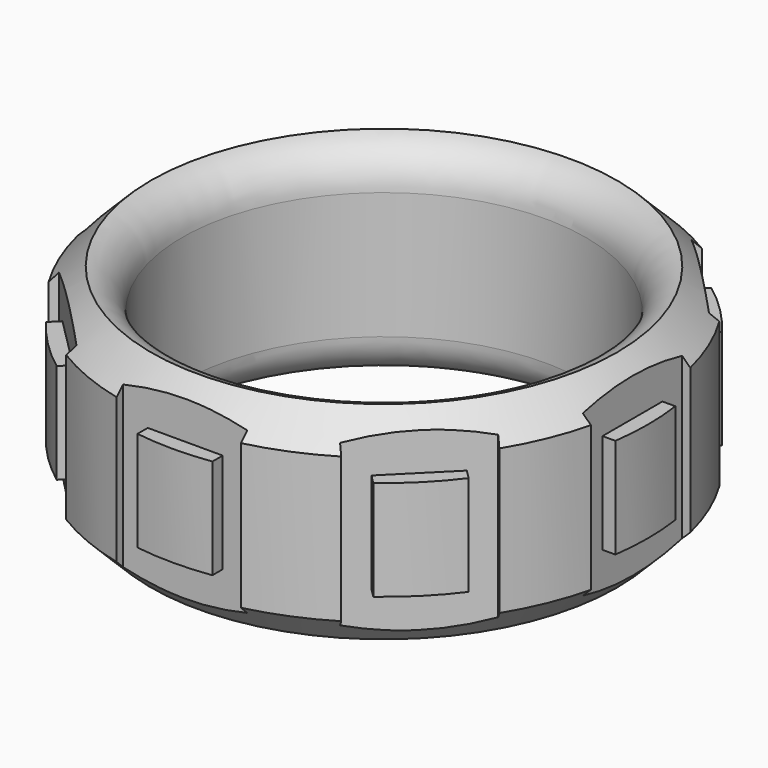
from build123d import *

# Parameters (mm, degrees)
F0_R            = 12.75
F0_R_2          = 9.75
F1_DEPTH        = 10
F2_SIZE         = 1.5
F4_W            = 6
F4_H            = 10
F4_W_2          = 3.618944902
F4_H_2          = 4.83566802
F5_DEPTH        = 2
F5_COPIES_COUNT = 8


# Not quite as in the source:
# - a fillet or chamfer that OpenCascade refuses, or shapes differently, is made with other operations: its cross-section is extruded or revolved along the edge and cut away or added
# - a pattern or mirror of a feature is missing from the dataset's text; its kind, count and spacing are read off the source's solid


with BuildPart() as f1:
    # F0 (on Top) → F1 (new body)
    with BuildSketch(Plane.XY):
        Circle(F0_R)
        Circle(F0_R_2, mode=Mode.SUBTRACT)
    extrude(amount=F1_DEPTH)

    # F2
    f2_edges = [f1.edges().sort_by_distance(p)[0] for p in [
        (-12.75, 0, 10),
        (-12.75, 0, 0),
    ]]
    chamfer(f2_edges, length=F2_SIZE)

    # F4 (on offset) → F5 (cut)
    with BuildSketch(Plane.YZ.offset(14)):
        with Locations((0, 5.0058439374)):
            Rectangle(F4_W, F4_H)
        with Locations((0, 5.0058439374)):
            Rectangle(F4_W_2, F4_H_2, mode=Mode.SUBTRACT)
    f5 = extrude(amount=-F5_DEPTH, mode=Mode.SUBTRACT)

    # F5_copies: F5 ×8 about axis
    f5_copies_axis = Axis((0, 0, 0), (0, 0, 1))
    for i in range(1, F5_COPIES_COUNT):
        add(f5.rotate(f5_copies_axis, i * 360 / F5_COPIES_COUNT), mode=Mode.SUBTRACT)

    # F6: fillet of radius 2 on 2 edges, made by hand

    # F6_s1 → F6_t2 (revolve, cut)
    with BuildSketch(Plane.XZ):
        with BuildLine():
            ThreePointArc((11.25, 10), (10.1688611699, 9.2882531983), (9.75, 8.0635083269))
            Line((9.75, 8.0635083269), (9.75, 10))
            Line((9.75, 10), (11.25, 10))
        make_face()
    revolve(axis=Axis((0, 0, 10), (0, 0, 1)), mode=Mode.SUBTRACT)

    # F6_s3 → F6_t4 (revolve, cut)
    with BuildSketch(Plane.XZ):
        with BuildLine():
            ThreePointArc((11.25, 0), (10.1688611699, 0.7117468017), (9.75, 1.9364916731))
            Line((9.75, 1.9364916731), (9.75, 0))
            Line((9.75, 0), (11.25, 0))
        make_face()
    revolve(axis=Axis((0, 0, 0), (0, 0, 1)), mode=Mode.SUBTRACT)


solid = f1.part
